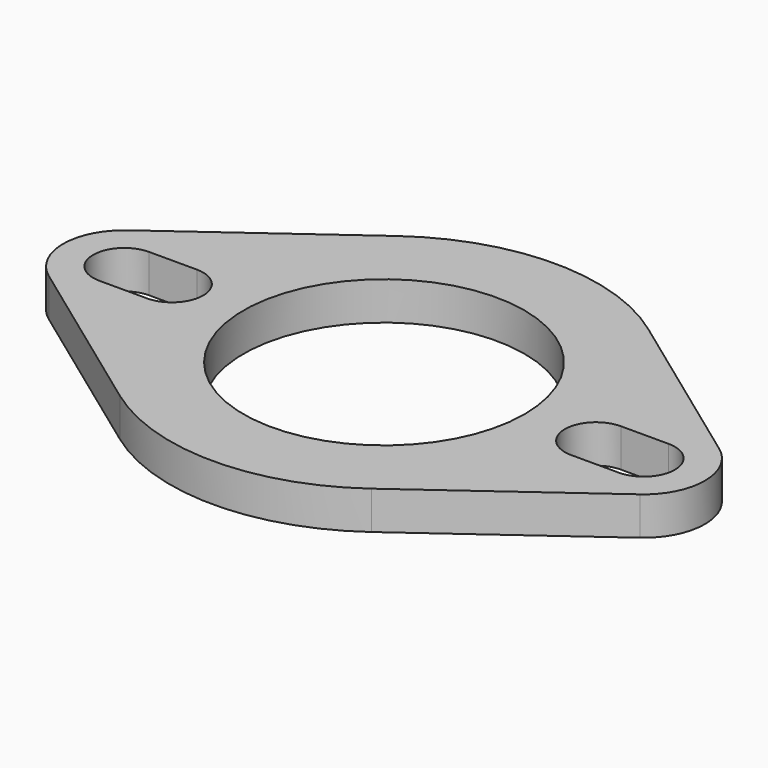
from build123d import *

# Parameters (mm, degrees)
F0_R     = 29.21
F1_DEPTH = 7.9375


# Not quite as in the source:
# - a length typed as a fraction of an inch, garbled in the dataset ("3 / 203.2 mm" for 3/8 in), is restored


with BuildPart() as f1:
    # F0 (on Top) → F1 (new body)
    with BuildSketch(Plane.XY):
        with BuildLine():
            Line((-61.4455882353, -10.2703608222), (-26.1470588235, -35.9462628778))
            ThreePointArc((-26.1470588235, -35.9462628778), (0, -44.45), (26.1470588235, -35.9462628778))
            Line((26.1470588235, -35.9462628778), (61.4455882353, -10.2703608222))
            ThreePointArc((61.4455882353, -10.2703608222), (66.675, 0), (61.4455882353, 10.2703608222))
            Line((61.4455882353, 10.2703608222), (26.1470588235, 35.9462628778))
            ThreePointArc((26.1470588235, 35.9462628778), (0, 44.45), (-26.1470588235, 35.9462628778))
            Line((-26.1470588235, 35.9462628778), (-61.4455882353, 10.2703608222))
            ThreePointArc((-61.4455882353, 10.2703608222), (-66.675, 0), (-61.4455882353, -10.2703608222))
        make_face()
        with BuildLine():
            ThreePointArc((-44.069, 6.477), (-37.592, 0), (-44.069, -6.477))
            Line((-44.069, -6.477), (-53.975, -6.477))
            ThreePointArc((-53.975, -6.477), (-60.452, 0), (-53.975, 6.477))
            Line((-53.975, 6.477), (-44.069, 6.477))
        make_face(mode=Mode.SUBTRACT)
        Circle(F0_R, mode=Mode.SUBTRACT)
        with BuildLine():
            ThreePointArc((44.069, -6.477), (37.592, 0), (44.069, 6.477))
            Line((44.069, 6.477), (53.975, 6.477))
            ThreePointArc((53.975, 6.477), (60.452, 0), (53.975, -6.477))
            Line((53.975, -6.477), (44.069, -6.477))
        make_face(mode=Mode.SUBTRACT)
    extrude(amount=F1_DEPTH)


solid = f1.part
